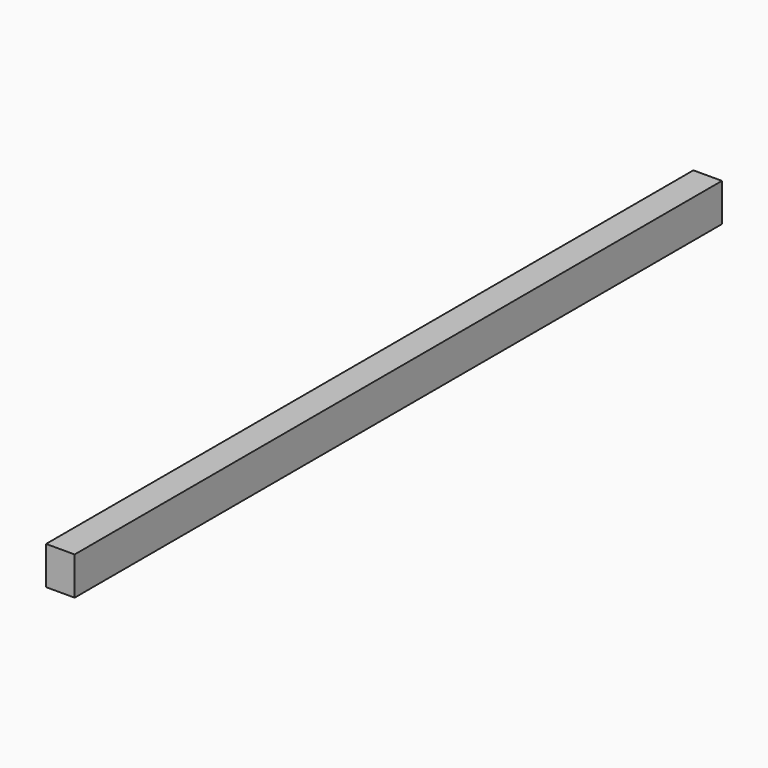
from build123d import *

# Parameters (mm, degrees)
F0_W     = 76.2
F0_H     = 101.6
F1_DEPTH = 2159


# Not quite as in the source:
# - the program builds the solid bodies; features that only make, move or delete a surface that nothing else refers to are left out


with BuildPart() as f1:
    # F0 (on Front) → F1 (new body)
    with BuildSketch(Plane.XZ):
        with Locations((38.1, 50.8)):
            Rectangle(F0_W, F0_H)
    extrude(amount=F1_DEPTH)


solid = f1.part
